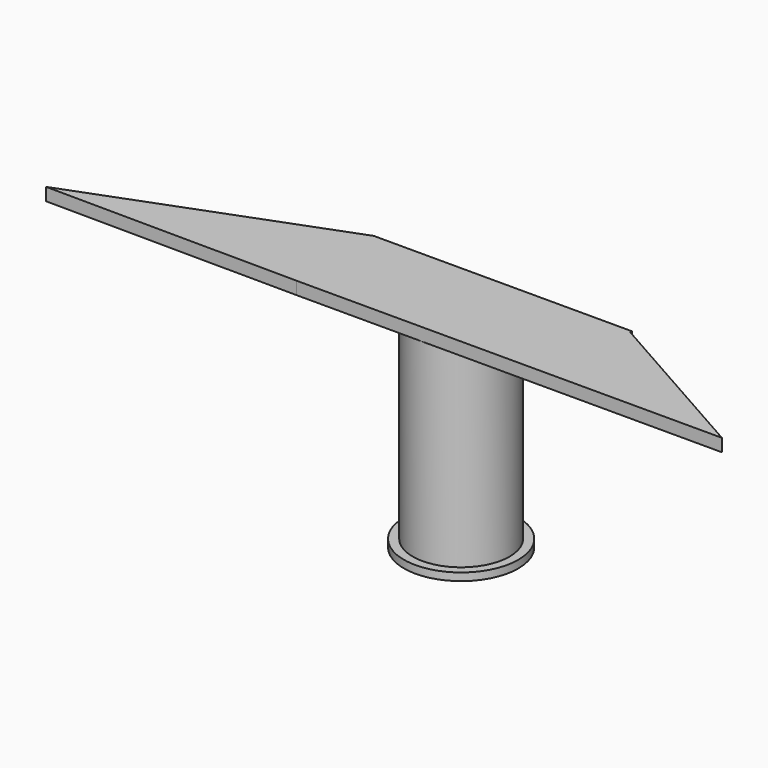
from build123d import *

# Parameters (mm, degrees)
F0_R     = 19.05
F1_DEPTH = 76.2
F2_W     = 101.6
F2_H     = 38.1
F3_DEPTH = 5
F4_R     = 22.479
F4_R_2   = 19.05
F5_DEPTH = 3
F6_R     = 12.7
F7_DEPTH = 3
F9_DEPTH = 5


with BuildPart() as f1:
    # F0 (on Top) → F1 (new body)
    with BuildSketch(Plane.XY):
        Circle(F0_R)
    extrude(amount=F1_DEPTH)

    # F2 (on face) → F3 (join)
    with BuildSketch(Plane.XY.offset(76.2)):
        with Locations((1.4545911372, -0.3322677247)):
            Rectangle(F2_W, F2_H)
    extrude(amount=F3_DEPTH)

    # F4 (on face) → F5 (join)
    with BuildSketch(Plane(origin=(0, 0, 0), x_dir=(1, 0, 0), z_dir=(0, 0, -1))):
        Circle(F4_R)
        Circle(F4_R_2, mode=Mode.SUBTRACT)
        Circle(F4_R_2)
    extrude(amount=F5_DEPTH)

    # F6 (on face) → F7 (join)
    with BuildSketch(Plane(origin=(0, 0, -3), x_dir=(1, 0, 0), z_dir=(0, 0, -1))):
        Circle(F6_R)
    extrude(amount=F7_DEPTH)

    # F8 (on face) → F9 (join)
    with BuildSketch(Plane.XY.offset(81.2)):
        Polygon((-49.3454088628, -19.3822677247), (-49.3454088628, 18.7177322753), (-148.3056545258, -18.6870153993), align=None)
        Polygon((118.0756762624, -19.3822677247), (52.2545911372, 17.8529117256), (52.2545911372, -19.3822677247), align=None)
    extrude(amount=-F9_DEPTH)


solid = f1.part
